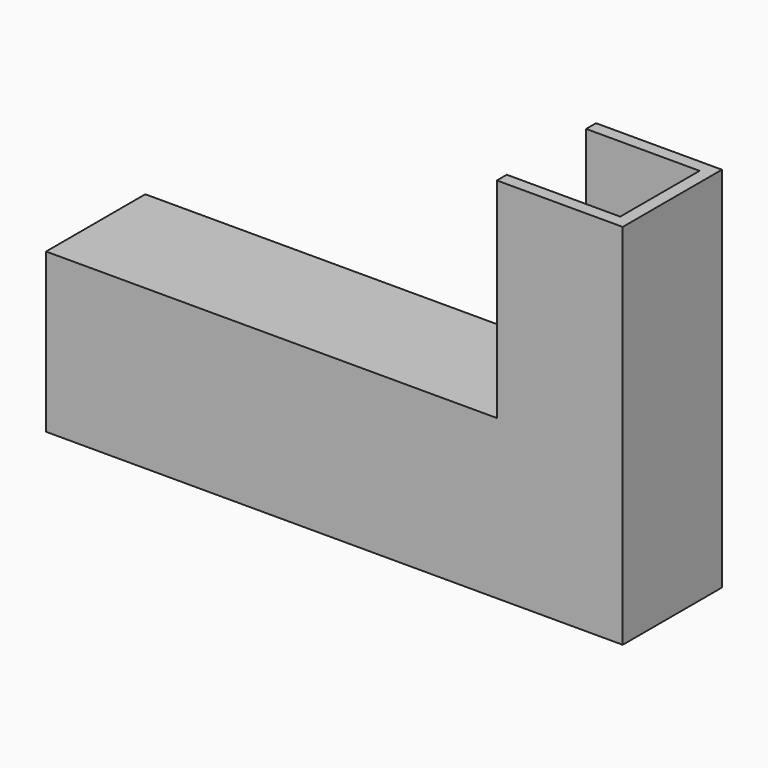
from build123d import *

# Parameters (mm, degrees)
F0_W     = 25.7852114737
F0_H     = 17.4429379404
F1_DEPTH = 25.4
F2_DEPTH = 25.4
F3_T     = 2.54


# Not quite as in the source:
# - a shell that OpenCascade refuses in one call is made with other operations: the cavity is built on its own and cut out


with BuildPart() as f1:
    # F0 (on Front) → F1 (new body)
    with BuildSketch(Plane.XZ):
        Polygon((36.1182577908, 32.5159132481), (-56.2155582011, 32.5159132481), (-56.2155582011, 0), (61.9034692645, 0), (61.9034692645, 32.5159132481), align=None)
        with Locations((49.0108635277, 41.2373822182)):
            Rectangle(F0_W, F0_H)
    extrude(amount=F1_DEPTH)

    # F2 (add): a face of the model
    f2_faces = [f1.faces().sort_by_distance(p)[0] for p in [
        (49.0108635277, -12.7, 49.9588511884),
    ]]
    extrude(f2_faces, amount=F2_DEPTH)

    # F3: shell of thickness 2.54, made by hand


with BuildPart() as f3_core1:
    # F3_t2: copy of F1
    add(f1.part)

    # the walls: a layer under each face that stays
    f3_faces = [f3_core1.faces().sort_by_distance(p)[0] for p in [
        (-10.0486502051, -12.7, 32.5159132481),
        (-36.5290536235, -25.4, 12.5598085314),
        (61.9034692645, -12.7, 37.6794255942),
        (2.8439555317, -12.7, 0),
        (-36.5290536235, 0, 12.5598085314),
        (-56.2155582011, -12.7, 16.257956624),
    ]]
    thicken(f3_faces, amount=-F3_T, mode=Mode.SUBTRACT)


with BuildPart() as f1_1:
    add(f1.part)

    # what is left inside the walls is the cavity
    f3_cavity = [f3_core1.part.solids().sort_by_distance(p)[0] for p in [
        (2.843956, -2.5654, 26.81295),
    ]]
    add(f3_cavity, mode=Mode.SUBTRACT)


solid = f1_1.part
